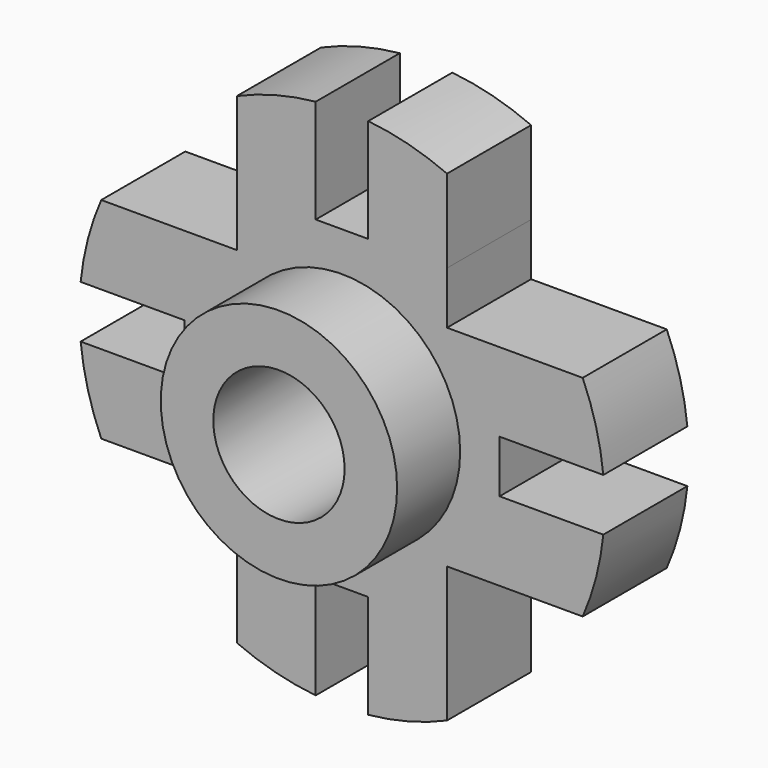
from build123d import *

# Parameters (mm, degrees)
F0_R     = 28.575
F1_DEPTH = 25.4
F0_R_2   = 15.875
F2_DEPTH = 44.45


# Not quite as in the source:
# - a feature names something its author has since deleted; it is built from what else it names


with BuildPart() as f1:
    # F0 (on Front) → F1 (new body)
    with BuildSketch(Plane.XZ):
        with BuildLine():
            Line((58.1987113259, 25.4), (38.1, 25.4))
            Line((38.1, 25.4), (38.1, 6.35))
            Line((38.1, 6.35), (63.1817022563, 6.35))
            ThreePointArc((63.1817022563, 6.35), (61.4331085437, 16.069324026), (58.1987113259, 25.4))
        make_face()
        with BuildLine():
            Line((63.1817022563, -6.35), (38.1, -6.35))
            Line((38.1, -6.35), (38.1, -25.4))
            Line((38.1, -25.4), (58.1987113259, -25.4))
            ThreePointArc((58.1987113259, -25.4), (61.4331085437, -16.069324026), (63.1817022563, -6.35))
        make_face()
        with BuildLine():
            Line((25.4, -58.1987113259), (25.4, -38.1))
            Line((25.4, -38.1), (6.35, -38.1))
            Line((6.35, -38.1), (6.35, -63.1817022563))
            ThreePointArc((6.35, -63.1817022563), (16.069324026, -61.4331085437), (25.4, -58.1987113259))
        make_face()
        with BuildLine():
            Line((-6.35, -63.1817022563), (-6.35, -38.1))
            Line((-6.35, -38.1), (-25.4, -38.1))
            Line((-25.4, -38.1), (-25.4, -58.1987113259))
            ThreePointArc((-25.4, -58.1987113259), (-16.069324026, -61.4331085437), (-6.35, -63.1817022563))
        make_face()
        with BuildLine():
            Line((-38.1, -25.4), (-38.1, -6.35))
            Line((-38.1, -6.35), (-63.1817022563, -6.35))
            ThreePointArc((-63.1817022563, -6.35), (-61.4331085437, -16.069324026), (-58.1987113259, -25.4))
            Line((-58.1987113259, -25.4), (-38.1, -25.4))
        make_face()
        with BuildLine():
            Line((6.35, 38.1), (25.4, 38.1))
            Line((25.4, 38.1), (25.4, 58.1987113259))
            ThreePointArc((25.4, 58.1987113259), (16.069324026, 61.4331085437), (6.35, 63.1817022563))
            Line((6.35, 63.1817022563), (6.35, 38.1))
        make_face()
        with BuildLine():
            Line((-25.4, 38.1), (-6.35, 38.1))
            Line((-6.35, 38.1), (-6.35, 63.1817022563))
            ThreePointArc((-6.35, 63.1817022563), (-16.069324026, 61.4331085437), (-25.4, 58.1987113259))
            Line((-25.4, 58.1987113259), (-25.4, 38.1))
        make_face()
        Polygon((25.3924280405, 25.4), (25.4, 38.1), (6.35, 38.1), (-6.35, 38.1), (-25.4, 38.1), (-25.4, 25.4), (-38.1, 25.4), (-38.1, 13.6643098667), (-38.1, 6.35), (-38.1, -6.35), (-38.1, -25.4), (-25.4, -25.4357550293), (-25.4, -38.1), (-6.35, -38.1), (6.35, -38.1), (25.4, -38.1), (25.4, -25.4), (38.1, -25.4), (38.1, -6.35), (38.1, 6.35), (38.1, 25.4), align=None)
        Circle(F0_R, mode=Mode.SUBTRACT)
        with BuildLine():
            Line((-38.1, 13.6643098667), (-38.1, 25.4))
            Line((-38.1, 25.4), (-58.1987113259, 25.4))
            ThreePointArc((-58.1987113259, 25.4), (-61.4331085437, 16.069324026), (-63.1817022563, 6.35))
            Line((-63.1817022563, 6.35), (-38.1, 6.35))
            Line((-38.1, 6.35), (-38.1, 13.6643098667))
        make_face()
    extrude(amount=F1_DEPTH)


with BuildPart() as f2:
    # F0 (on Front) → F2 (new body)
    with BuildSketch(Plane.XZ):
        Circle(F0_R)
        Circle(F0_R_2, mode=Mode.SUBTRACT)
    extrude(amount=F2_DEPTH)


solid = Compound([f1.part, f2.part])
